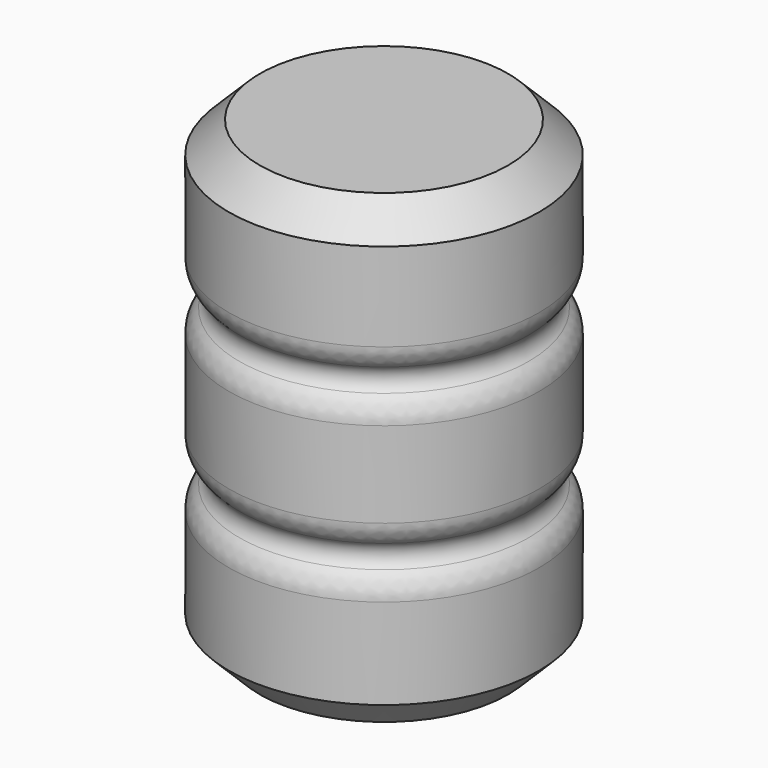
from build123d import *

# Parameters (mm, degrees)
F2_SIZE = 5.08
F3_R    = 5.08


with BuildPart() as f1:
    # F0 (on Front) → F1 (revolve)
    with BuildSketch(Plane.XZ):
        with BuildLine():
            Line((-25.4, 0), (0, 0))
            Line((0, 0), (0, 23.0479238248))
            ThreePointArc((0, 23.0479238248), (-2.54, 25.5879238248), (0, 28.1279238248))
            Line((0, 28.1279238248), (0, 48.4448967195))
            ThreePointArc((0, 48.4448967195), (-2.54, 50.9848967195), (0, 53.5248967195))
            Line((0, 53.5248967195), (0, 76.2))
            Line((0, 76.2), (-25.4, 76.2))
            Line((-25.4, 76.2), (-25.4, 0))
        make_face()
    revolve(axis=Axis((-25.4, 0, 38.1), (0, 0, 1)))

    # F2
    f2_edges = [f1.edges().sort_by_distance(p)[0] for p in [
        (-50.8, 0, 76.2),
        (-50.8, 0, 0),
    ]]
    chamfer(f2_edges, length=F2_SIZE)

    # F3
    f3_edges = [f1.edges().sort_by_distance(p)[0] for p in [
        (-50.8, 0, 53.524897),
        (-50.8, 0, 28.127924),
        (-50.8, 0, 23.047924),
        (-50.8, 0, 48.444897),
    ]]
    fillet(f3_edges, radius=F3_R)


solid = f1.part
